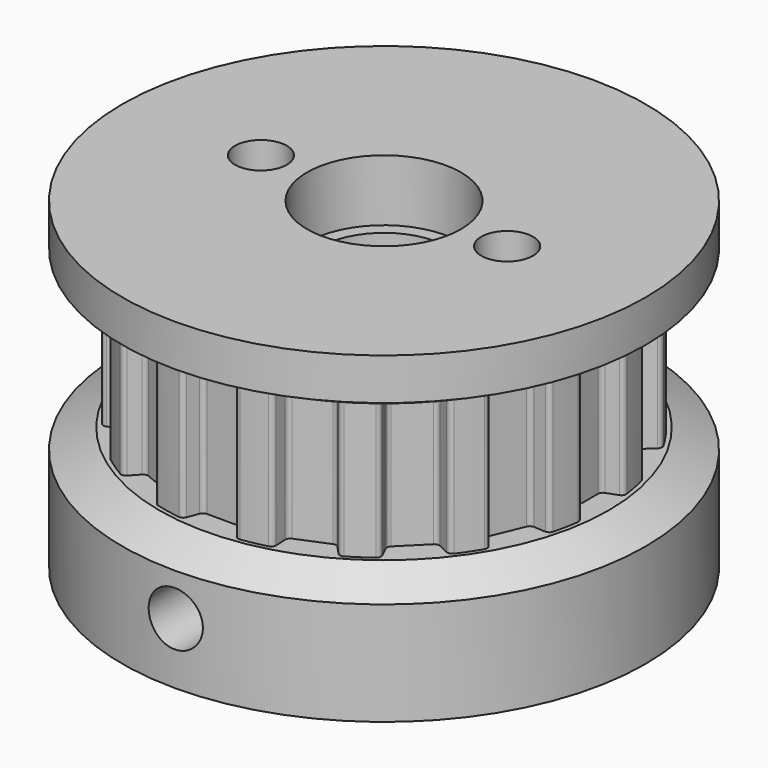
from build123d import *

# Parameters (mm, degrees)
F0_R            = 26.9875
F1_DEPTH        = 12.7
F2_R            = 22.733
F3_DEPTH        = 14.224
F5_DEPTH        = 14.224
F5_COPIES_COUNT = 16
F7_R            = 6.604
F8_DEPTH        = 26.925
F9_R            = 1.651
F10_DEPTH       = 19.05
F13_DEPTH       = 4.572
F14_R           = 2.794
F15_DEPTH       = 9.652
F15_DEPTH_BACK  = 25.4
F16_SIZE2       = 2.032
F16_SIZE        = 3.81
F18_R           = 26.9875
F18_R_2         = 2.667
F18_R_3         = 7.9375
F19_DEPTH       = 6.35


# Not quite as in the source:
# - a fillet or chamfer that OpenCascade refuses, or shapes differently, is made with other operations: its cross-section is extruded or revolved along the edge and cut away or added
# - a pattern or mirror of a feature is missing from the dataset's text; its kind, count and spacing are read off the source's solid


with BuildPart() as f1:
    # F0 (on Top) → F1 (new body)
    with BuildSketch(Plane.XY):
        Circle(F0_R)
    extrude(amount=F1_DEPTH)

    # F2 (on face) → F3 (join)
    with BuildSketch(Plane.XY.offset(12.7)):
        Circle(F2_R)
    extrude(amount=F3_DEPTH)

    # F4 (on face) → F5 (cut, through all)
    with BuildSketch(Plane.XY.offset(26.924)):
        with BuildLine():
            ThreePointArc((3.1576449696, 22.5126312822), (2.39e-08, 22.733), (-3.1576449222, 22.5126312888))
            ThreePointArc((-3.1576449222, 22.5126312888), (-2.8253839703, 22.4449607994), (-2.6097192194, 22.1833019556))
            Line((-2.6097192194, 22.1833019556), (-2.1918638514, 21.0352537672))
            ThreePointArc((-2.1918638514, 21.0352537672), (-2.0058768297, 20.7928707615), (-1.7145, 20.701))
            Line((-1.7145, 20.701), (1.7145, 20.701))
            ThreePointArc((1.7145, 20.701), (2.0058768297, 20.7928707615), (2.1918638514, 21.0352537672))
            Line((2.1918638514, 21.0352537672), (2.6097192194, 22.1833019556))
            ThreePointArc((2.6097192194, 22.1833019556), (2.8253839908, 22.4449608118), (3.1576449696, 22.5126312822))
        make_face()
    f5 = extrude(amount=-F5_DEPTH, mode=Mode.SUBTRACT)

    # F5_copies: F5 ×16 about axis
    f5_copies_axis = Axis((0, 0, 0), (0, 0, 1))
    for i in range(1, F5_COPIES_COUNT):
        add(f5.rotate(f5_copies_axis, i * 360 / F5_COPIES_COUNT), mode=Mode.SUBTRACT)

    # F7 (on face) → F8 (cut, through all)
    with BuildSketch(Plane(origin=(0, 0, 0), x_dir=(1, 0, 0), z_dir=(0, 0, -1))):
        Circle(F7_R)
    extrude(amount=-F8_DEPTH, mode=Mode.SUBTRACT)

    # F9 (on face) → F10 (cut)
    with BuildSketch(Plane.XY.offset(26.924)):
        with Locations((-12.7, 0)):
            Circle(F9_R)
        with Locations((12.7, 0)):
            Circle(F9_R)
    extrude(amount=-F10_DEPTH, mode=Mode.SUBTRACT)

    # F12 (on offset) → F13 (cut)
    with BuildSketch(Plane.XZ.offset(14.224)):
        Polygon((-5.461, 0), (5.461, 0), (5.461, 3.15290982), (5.461, 9.4587294601), (0, 14.9197294601), (-5.461, 9.4587294601), (-5.461, 3.15290982), align=None)
    extrude(amount=-F13_DEPTH, mode=Mode.SUBTRACT)

    # F14 (on face) → F15 (cut, two sides)
    with BuildSketch(Plane.XZ.offset(9.652)) as f15_sk:
        with Locations((0, 6.3058196401)):
            Circle(F14_R)
    extrude(amount=-F15_DEPTH, mode=Mode.SUBTRACT)
    extrude(f15_sk.sketch, amount=F15_DEPTH_BACK, mode=Mode.SUBTRACT)

    # F16
    f16_edges = [f1.edges().sort_by_distance(p)[0] for p in [
        (-26.9875, 0, 12.7),
    ]]
    f16_side = f1.faces().sort_by_distance((-26.224178, 0, 12.7))[0]
    chamfer(f16_edges, length=F16_SIZE, length2=F16_SIZE2, reference=f16_side)


with BuildPart() as f19:
    # F18 (on offset) → F19 (new body, through all)
    with BuildSketch(Plane.XY.offset(33.274)):
        Circle(F18_R)
        with Locations((-12.7, 0)):
            Circle(F18_R_2, mode=Mode.SUBTRACT)
        Circle(F18_R_3, mode=Mode.SUBTRACT)
        with Locations((12.7, 0)):
            Circle(F18_R_2, mode=Mode.SUBTRACT)
    extrude(amount=-F19_DEPTH)

    # F20: chamfer of 3.81 x 2.032 on 1 edges, made by hand

    # F20_s1 → F20_t2 (revolve, cut)
    with BuildSketch(Plane.XZ):
        Polygon((26.9875, 28.956), (23.1775, 26.924), (26.9875, 26.924), align=None)
    revolve(axis=Axis((0, 0, 26.924), (0, 0, 1)), mode=Mode.SUBTRACT)


solid = Compound([f1.part, f19.part])
